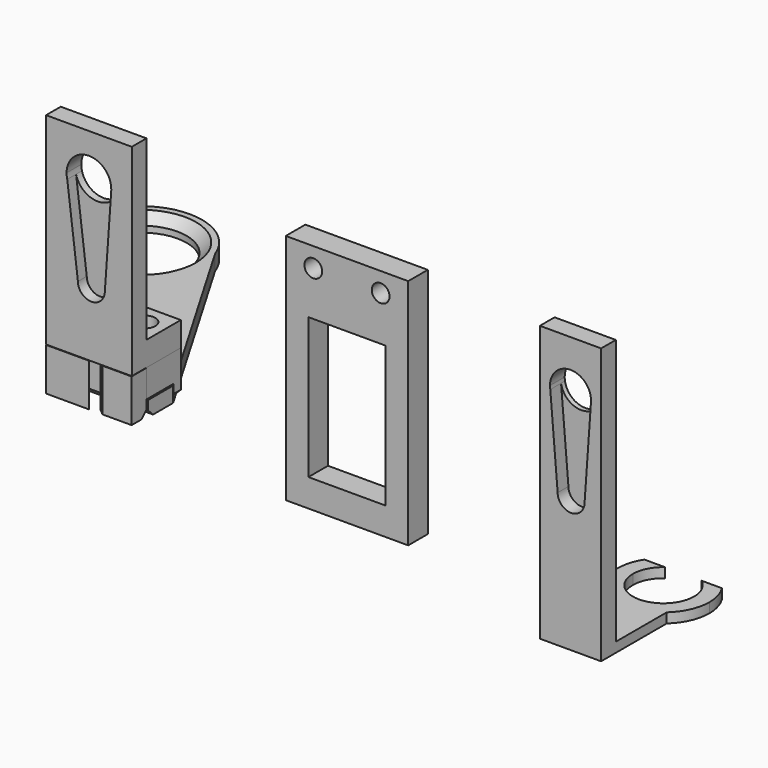
from build123d import *

# Parameters (mm, degrees)
F0_W           = 20
F0_H           = 38
F0_W_2         = 12.6
F0_H_2         = 23
F0_R           = 1.45
F1_DEPTH       = 4
F2_W           = 10
F2_H           = 43.4
F2_H_2         = 1.6
F3_DEPTH       = 3
F4_DEPTH       = 0.8
F5_DEPTH       = 20
F7_DEPTH       = 1.6
F8_DEPTH       = 25
F9_W           = 14
F9_H           = 28.9722495526
F10_DEPTH      = 3
F11_DEPTH      = 1.2
F9_H_2         = 5.0277504474
F9_H_3         = 2
F12_DEPTH      = 7
F9_H_4         = 4
F13_DEPTH      = 3
F13_DEPTH_BACK = 7
F14_R          = 1.8
F14_R_2        = 1.45
F15_DEPTH      = 25
F16_DEPTH      = 9
F18_START      = -15
F17_R          = 7.5
F18_DEPTH      = 2.5
F19_SIZE       = 1.5
F20_T1_DEPTH   = 17.1433659759
F20_T6_DEPTH   = 7.7573358308
F20_T11_DEPTH  = 6.5816100927
F22_START      = -10.5
F22_DEPTH      = 7
F23_SIZE       = 0.99999
F24_R          = 2.85
F24_R_2        = 1.5
F25_DEPTH      = 1.8
F26_DEPTH      = 25


# Not quite as in the source:
# - a fillet or chamfer that OpenCascade refuses, or shapes differently, is made with other operations: its cross-section is extruded or revolved along the edge and cut away or added
# - a fillet or chamfer is up to 0.001 mm smaller than in the source, because OpenCascade refuses the exact size
# - ends of sketch curves that miss each other by under 0.0002 mm in the source are joined


with BuildPart() as f1:
    # F0 (on Front) → F1 (new body)
    with BuildSketch(Plane.XZ):
        with Locations((0, -0.4293409586)):
            Rectangle(F0_W, F0_H)
        with Locations((0, -3.4033237249)):
            Rectangle(F0_W_2, F0_H_2, mode=Mode.SUBTRACT)
        with Locations((-5.5, 15.3828505427)):
            Circle(F0_R, mode=Mode.SUBTRACT)
        with Locations((5.5, 15.3828505427)):
            Circle(F0_R, mode=Mode.SUBTRACT)
    extrude(amount=F1_DEPTH)


with BuildPart() as f3:
    # F2 (on Front) → F3 (new body)
    with BuildSketch(Plane.XZ):
        with Locations((35.7141409814, -3.2186261386)):
            Rectangle(F2_W, F2_H)
        with BuildLine():
            ThreePointArc((32.3641409814, 10.4278577492), (35.7141409814, 13.7778577492), (39.0641409814, 10.4278577492))
            Line((39.0641409814, 10.4278577492), (39.0724650475, 10.4278577492))
            Line((39.0724650475, 10.4278577492), (39.055837541, 10.1921373555))
            Line((39.055837541, 10.1921373555), (38.0143784106, -4.5721422508))
            ThreePointArc((38.0143784106, -4.5721422508), (35.8143784106, -6.7721422508), (33.6143784106, -4.5721422508))
            Line((33.6143784106, -4.5721422508), (32.4103653119, 9.8732711234))
            ThreePointArc((32.4103653119, 9.8732711234), (32.3757170649, 10.1496029135), (32.3641409814, 10.4278577492))
        make_face(mode=Mode.SUBTRACT)
        with Locations((35.7141409814, -25.7186261386)):
            Rectangle(F2_W, F2_H_2)
    extrude(amount=F3_DEPTH)

    # F2 (on Front) → F4 (join)
    with BuildSketch(Plane.XZ):
        with Locations((35.7141409814, -3.2186261386)):
            Rectangle(F2_W, F2_H)
        with BuildLine():
            ThreePointArc((32.3641409814, 10.4278577492), (35.7141409814, 13.7778577492), (39.0641409814, 10.4278577492))
            Line((39.0641409814, 10.4278577492), (39.0724650475, 10.4278577492))
            Line((39.0724650475, 10.4278577492), (39.055837541, 10.1921373555))
            Line((39.055837541, 10.1921373555), (38.0143784106, -4.5721422508))
            ThreePointArc((38.0143784106, -4.5721422508), (35.8143784106, -6.7721422508), (33.6143784106, -4.5721422508))
            Line((33.6143784106, -4.5721422508), (32.4103653119, 9.8732711234))
            ThreePointArc((32.4103653119, 9.8732711234), (32.3757170649, 10.1496029135), (32.3641409814, 10.4278577492))
        make_face(mode=Mode.SUBTRACT)
        with BuildLine():
            Line((38.0143784106, -4.5721422508), (39.055837541, 10.1921373555))
            ThreePointArc((39.055837541, 10.1921373555), (35.8746975664, 7.0817074861), (32.4103653119, 9.8732711234))
            Line((32.4103653119, 9.8732711234), (33.6143784106, -4.5721422508))
            ThreePointArc((33.6143784106, -4.5721422508), (35.8143784106, -2.3721422508), (38.0143784106, -4.5721422508))
        make_face()
        with BuildLine():
            Line((33.6143784106, -4.5721422508), (38.0143784106, -4.5721422508))
            ThreePointArc((38.0143784106, -4.5721422508), (35.8143784106, -2.3721422508), (33.6143784106, -4.5721422508))
        make_face()
        with BuildLine():
            ThreePointArc((33.6143784106, -4.5721422508), (35.8143784106, -6.7721422508), (38.0143784106, -4.5721422508))
            Line((38.0143784106, -4.5721422508), (33.6143784106, -4.5721422508))
        make_face()
    extrude(amount=F4_DEPTH)

    # F2 (on Front) → F5 (join)
    with BuildSketch(Plane.XZ):
        with Locations((35.7141409814, -25.7186261386)):
            Rectangle(F2_W, F2_H_2)
    extrude(amount=-F5_DEPTH)

    # F6 (on face) → F7 (join)
    with BuildSketch(Plane(origin=(0, 0, -26.5186261386), x_dir=(1, 0, 0), z_dir=(0, 0, -1))):
        with BuildLine():
            Line((30.7141409814, -15.9823000431), (30.7141409814, -20))
            Line((30.7141409814, -20), (32.7378844363, -20))
            ThreePointArc((32.7378844363, -20), (31.2486445239, -18.2316033447), (30.7141409814, -15.9823000431))
        make_face()
        with BuildLine():
            Line((38.6903921621, -20), (40.7141409814, -20))
            Line((40.7141409814, -20), (40.7141409814, -15.9823000431))
            ThreePointArc((40.7141409814, -15.9823000431), (40.1796320745, -18.2316033447), (38.6903921621, -20))
        make_face()
        with BuildLine():
            ThreePointArc((40.7141409814, -10.3921324984), (35.7141418978, -8.4823000431), (30.7141409814, -10.3921277003))
            Line((30.7141409814, -10.3921277003), (30.7141409814, -15.9823000431))
            ThreePointArc((30.7141409814, -15.9823000431), (35.7141382992, -10.9823000431), (40.7141382992, -15.9823000431))
            Line((40.7141382992, -15.9823000431), (40.7141409814, -10.3921324984))
        make_face()
        with BuildLine():
            Line((40.7141409814, -20), (42.0472328869, -20))
            ThreePointArc((42.0472328869, -20), (42.916506292, -18.0741641152), (43.2141382992, -15.9823000431))
            ThreePointArc((43.2141382992, -15.9823000431), (42.5606710026, -12.9204395071), (40.7141409814, -10.3921324984))
            Line((40.7141409814, -10.3921324984), (40.7141409814, -15.9823000431))
            Line((40.7141409814, -15.9823000431), (40.7141409814, -20))
        make_face()
        with BuildLine():
            ThreePointArc((30.7141409814, -10.3921277003), (28.2853062533, -14.9515457398), (29.3810437116, -20))
            Line((29.3810437116, -20), (30.7141409814, -20))
            Line((30.7141409814, -20), (30.7141409814, -15.9823000431))
            Line((30.7141409814, -15.9823000431), (30.7141409814, -10.3921277003))
        make_face()
    extrude(amount=-F7_DEPTH)

    # F6 (on face) → F8 (cut)
    with BuildSketch(Plane(origin=(0, 0, -26.5186261386), x_dir=(1, 0, 0), z_dir=(0, 0, -1))):
        with BuildLine():
            add(Edge.make_bspline(
                [(33.1693342328, -2.8546717949), (33.1693342328, -5.4527480063), (36.9193342328, -4.1537099006), (40.6693342328, -2.8546717949), (36.9193342328, -1.5556336892), (33.1693342328, -0.2565955836), (33.1693342328, -2.8546717949)],
                knots=[0, 0, 0, 2.0943951024, 2.0943951024, 4.1887902048, 4.1887902048, 6.2831853072, 6.2831853072, 6.2831853072], degree=2, weights=[1, 0.5, 1, 0.5, 1, 0.5, 1]))
        make_face()
        with BuildLine():
            ThreePointArc((40.7141382992, -15.9823000431), (35.7141382992, -10.9823000431), (30.7141382992, -15.9823000431))
            ThreePointArc((30.7141382992, -15.9823000431), (31.2486445239, -18.2316033447), (32.7378844363, -20))
            Line((32.7378844363, -20), (38.6903921621, -20))
            ThreePointArc((38.6903921621, -20), (40.1796320745, -18.2316033447), (40.7141382992, -15.9823000431))
        make_face()
    extrude(amount=-F8_DEPTH, mode=Mode.SUBTRACT)


with BuildPart() as f10:
    # F9 (on Front) → F10 (new body)
    with BuildSketch(Plane.XZ):
        with Locations((-42.9501784987, 8.0518015102)):
            Rectangle(F9_W, F9_H)
        with BuildLine():
            ThreePointArc((-46.6001784987, 15.3248970558), (-42.9501784987, 18.9748970558), (-39.3001784987, 15.3248970558))
            Line((-39.3001784987, 15.3248970558), (-39.2911089939, 15.3248970558))
            Line((-39.2911089939, 15.3248970558), (-39.3092255247, 15.0680674607))
            Line((-39.3092255247, 15.0680674607), (-40.3491956308, 0.3248970558))
            ThreePointArc((-40.3491956308, 0.3248970558), (-42.5491956308, -1.8751029442), (-44.7491956308, 0.3248970558))
            Line((-44.7491956308, 0.3248970558), (-46.4906866316, 14.4375965648))
            ThreePointArc((-46.4906866316, 14.4375965648), (-46.5727021139, 14.8778817791), (-46.6001784987, 15.3248970558))
        make_face(mode=Mode.SUBTRACT)
    extrude(amount=F10_DEPTH)

    # F9 (on Front) → F11 (join)
    with BuildSketch(Plane.XZ):
        with Locations((-42.9501784987, 8.0518015102)):
            Rectangle(F9_W, F9_H)
        with BuildLine():
            ThreePointArc((-46.6001784987, 15.3248970558), (-42.9501784987, 18.9748970558), (-39.3001784987, 15.3248970558))
            Line((-39.3001784987, 15.3248970558), (-39.2911089939, 15.3248970558))
            Line((-39.2911089939, 15.3248970558), (-39.3092255247, 15.0680674607))
            Line((-39.3092255247, 15.0680674607), (-40.3491956308, 0.3248970558))
            ThreePointArc((-40.3491956308, 0.3248970558), (-42.5491956308, -1.8751029442), (-44.7491956308, 0.3248970558))
            Line((-44.7491956308, 0.3248970558), (-46.4906866316, 14.4375965648))
            ThreePointArc((-46.4906866316, 14.4375965648), (-46.5727021139, 14.8778817791), (-46.6001784987, 15.3248970558))
        make_face(mode=Mode.SUBTRACT)
        with BuildLine():
            Line((-40.3491956308, 0.3248970558), (-39.3092255247, 15.0680674607))
            ThreePointArc((-39.3092255247, 15.0680674607), (-42.6309674726, 11.6888821603), (-46.4906866316, 14.4375965648))
            Line((-46.4906866316, 14.4375965648), (-44.7491956308, 0.3248970558))
            ThreePointArc((-44.7491956308, 0.3248970558), (-42.5491956308, 2.5248970558), (-40.3491956308, 0.3248970558))
        make_face()
        with BuildLine():
            Line((-44.7491956308, 0.3248970558), (-40.3491956308, 0.3248970558))
            ThreePointArc((-40.3491956308, 0.3248970558), (-42.5491956308, 2.5248970558), (-44.7491956308, 0.3248970558))
        make_face()
        with BuildLine():
            ThreePointArc((-44.7491956308, 0.3248970558), (-42.5491956308, -1.8751029442), (-40.3491956308, 0.3248970558))
            Line((-40.3491956308, 0.3248970558), (-44.7491956308, 0.3248970558))
        make_face()
    extrude(amount=F11_DEPTH)

    # F9 (on Front) → F13 (join, two sides)
    with BuildSketch(Plane.XZ) as f13_sk:
        with Locations((-42.9501784987, -8.4343232661)):
            Rectangle(F9_W, F9_H_4)
    extrude(amount=F13_DEPTH)
    extrude(f13_sk.sketch, amount=-F13_DEPTH_BACK)

    # F14 (on face) → F15 (cut)
    with BuildSketch(Plane.XY.offset(-6.4343232661)):
        with Locations((-39.2406210303, 3.6812750623)):
            Circle(F14_R)
        with Locations((-39.2406210303, 3.6812750623)):
            Circle(F14_R_2, mode=Mode.SUBTRACT)
        with Locations((-46.3644899428, 3.6812750623)):
            Circle(F14_R)
        with Locations((-46.3644899428, 3.6812750623)):
            Circle(F14_R_2, mode=Mode.SUBTRACT)
        with Locations((-39.2406210303, 3.6812750623)):
            Circle(F14_R_2)
        with Locations((-46.3644899428, 3.6812750623)):
            Circle(F14_R_2)
    extrude(amount=-F15_DEPTH, mode=Mode.SUBTRACT)


with BuildPart() as f12:
    # F9 (on Front) → F12 (new body)
    with BuildSketch(Plane.XZ):
        with Locations((-42.9501784987, -12.9481984898)):
            Rectangle(F9_W, F9_H_2)
        with Locations((-42.9501784987, -16.4620737135)):
            Rectangle(F9_W, F9_H_3)
    extrude(amount=-F12_DEPTH)

    # F14 (on face) → F16 (cut)
    with BuildSketch(Plane.XY.offset(-6.4343232661)):
        with Locations((-39.2406210303, 3.6812750623)):
            Circle(F14_R_2)
        with Locations((-46.3644899428, 3.6812750623)):
            Circle(F14_R_2)
    extrude(amount=-F16_DEPTH, mode=Mode.SUBTRACT)

    # F17 (on Top) → F18 (join)
    with BuildSketch(Plane.XY.offset(F18_START)):
        with BuildLine():
            ThreePointArc((-70.2937416126, 25.9747048099), (-59.5394972596, 24.2841557658), (-53.6139108759, 33.416469475))
            ThreePointArc((-53.6139108759, 33.416469475), (-53.7632412512, 35.1381860441), (-54.2067724648, 36.8084816969))
            ThreePointArc((-54.2067724648, 36.8084816969), (-69.1998067035, 41.7109114576), (-70.2937416126, 25.9747048099))
        make_face()
        with Locations((-63.6139108759, 33.416469475)):
            Circle(F17_R, mode=Mode.SUBTRACT)
        with BuildLine():
            ThreePointArc((-54.2067724648, 36.8084816969), (-53.7632412512, 35.1381860441), (-53.6139108759, 33.416469475))
            ThreePointArc((-53.6139108759, 33.416469475), (-59.5394972596, 24.2841557658), (-70.2937416126, 25.9747048099))
            Line((-70.2937416126, 25.9747048099), (-47.673817724, 0))
            Line((-47.673817724, 0), (-35.673817724, 0))
            Line((-35.673817724, 0), (-35.673817724, 5.0887558609))
            Line((-35.673817724, 5.0887558609), (-54.2067724648, 36.8084816969))
        make_face()
    extrude(amount=-F18_DEPTH)

    # F19
    f19_edges = [f12.edges().sort_by_distance(p)[0] for p in [
        (-71.113911, 33.416469, -15),
    ]]
    chamfer(f19_edges, length=F19_SIZE)

    # F20: chamfer of 1 on 3 edges, made by hand

    # F20_s2 → F20_t1 (cut)
    with BuildSketch(Plane.YZ.offset(-50.245500712)):
        Polygon((1, -17.5), (0, -16.5), (0, -17.5), align=None)
    extrude(amount=F20_T1_DEPTH, mode=Mode.SUBTRACT)


with BuildPart() as f20_tool4:
    # F20_s5 → F20_t6 (new body)
    with BuildSketch(Plane.XZ.offset(2.571682988)):
        Polygon((-49.9501784987, -16.4620737135), (-48.9501784987, -17.4620737135), (-49.9501784987, -17.4620737135), align=None)
    extrude(amount=-F20_T6_DEPTH)

    split(bisect_by=Plane(origin=(-27.1125092059, -23.6107743728, 0), x_dir=(0, 0, 1), z_dir=(-0.7541276951, -0.6567278123, 0)), keep=Keep.TOP)


with BuildPart() as f12_1:
    add(f12.part)

    # F20_t3: cut F20_tool4
    add(f20_tool4.part, mode=Mode.SUBTRACT)


with BuildPart() as f20_tool9:
    # F20_s10 → F20_t11 (new body)
    with BuildSketch(Plane.XZ.offset(-2.9900728953)):
        Polygon((-35.9501784987, -16.4620737135), (-36.9501784987, -17.4620737135), (-35.9501784987, -17.4620737135), align=None)
    extrude(amount=-F20_T11_DEPTH)

    split(bisect_by=Plane(origin=(-24.3784345493, -14.2436421579, 0), x_dir=(0, 0, 1), z_dir=(0.8634258622, 0.5044757482, 0)), keep=Keep.TOP)


with BuildPart() as f12_2:
    add(f12_1.part)

    # F20_t8: cut F20_tool9
    add(f20_tool9.part, mode=Mode.SUBTRACT)

    # F21 (on Top) → F22 (join)
    with BuildSketch(Plane.XY.offset(F22_START)):
        Polygon((-48.912383616, 0), (-49.9247312546, 0), (-49.9247312546, -3), (-42.9510335326, -3), (-44.3568192422, -2.1385268774), (-48.912383616, -2.1385268774), align=None)
        Polygon((-41.7726673186, -2.1385268774), (-40.7336801291, -3), (-35.9773358107, -3), (-35.9773358107, 0), (-36.9773358107, 0), (-36.9773358107, -2.1385268774), align=None)
    extrude(amount=-F22_DEPTH)

    # F23 (size 1 in the source; OpenCascade refuses exactly that, so slightly less here)
    f23_edges = [f12_2.edges().sort_by_distance(p)[0] for p in [
        (-36.477336, 0, -17.5),
        (-49.418557, 0, -17.5),
    ]]
    chamfer(f23_edges, length=F23_SIZE)

    # F24 (on face) → F25 (cut)
    with BuildSketch(Plane(origin=(0, 0, -17.5), x_dir=(1, 0, 0), z_dir=(0, 0, -1))):
        with Locations((-51.1756800115, -10.2872671559)):
            Circle(F24_R)
        with Locations((-51.1756800115, -10.2872671559)):
            Circle(F24_R_2, mode=Mode.SUBTRACT)
        with Locations((-43.1130826473, -10.2872671559)):
            Circle(F24_R)
        with Locations((-43.1130826473, -10.2872671559)):
            Circle(F24_R_2, mode=Mode.SUBTRACT)
    extrude(amount=-F25_DEPTH, mode=Mode.SUBTRACT)

    # F24 (on face) → F26 (cut)
    with BuildSketch(Plane(origin=(0, 0, -17.5), x_dir=(1, 0, 0), z_dir=(0, 0, -1))):
        with Locations((-51.1756800115, -10.2872671559)):
            Circle(F24_R_2)
        with Locations((-43.1130826473, -10.2872671559)):
            Circle(F24_R_2)
    extrude(amount=-F26_DEPTH, mode=Mode.SUBTRACT)


solid = Compound([f1.part, f3.part, f10.part, f12_2.part])
